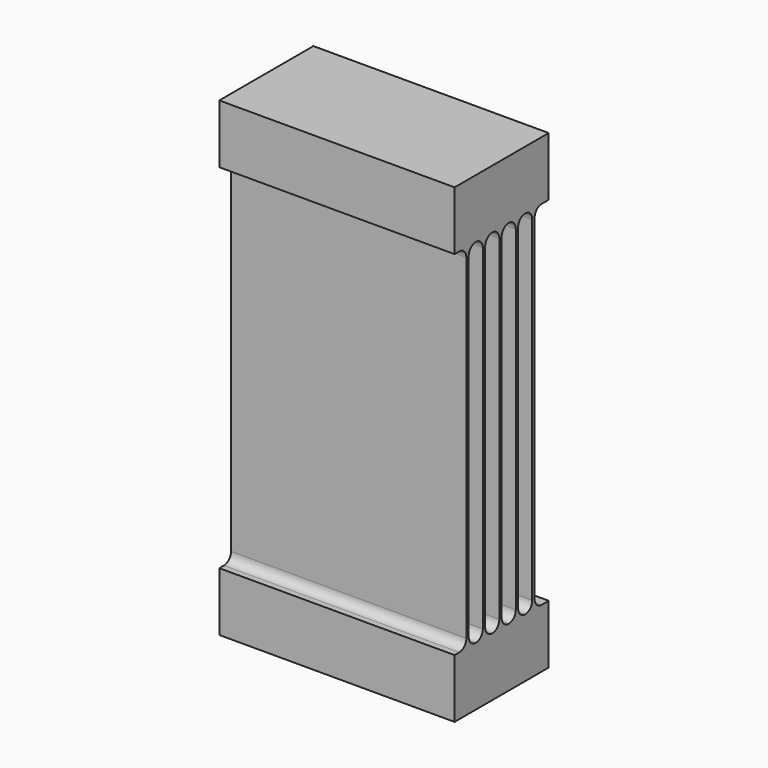
from build123d import *

# Parameters (mm, degrees)
F0_W     = 40
F0_H     = 20
F1_DEPTH = 10
F3_W     = 40
F3_H     = 0.5
F4_DEPTH = 30
F6_R     = 1.49999


# Not quite as in the source:
# - a fillet or chamfer is up to 0.001 mm smaller than in the source, because OpenCascade refuses the exact size


with BuildPart() as f1:
    # F0 (on Top) → F1 (new body)
    with BuildSketch(Plane.XY):
        with Locations((20, -10)):
            Rectangle(F0_W, F0_H)
    extrude(amount=F1_DEPTH)

    # F3 (on face) → F4 (join)
    with BuildSketch(Plane.XY.offset(10)):
        with Locations((20, -3.25)):
            Rectangle(F3_W, F3_H)
        with Locations((20, -6.75)):
            Rectangle(F3_W, F3_H)
        with Locations((20, -10.25)):
            Rectangle(F3_W, F3_H)
        with Locations((20, -13.75)):
            Rectangle(F3_W, F3_H)
        with Locations((20, -17.25)):
            Rectangle(F3_W, F3_H)
    extrude(amount=F4_DEPTH)

    # F5: F1 across face


with BuildPart() as f1_1:
    add(f1.part)
    add(f1.part.mirror(Plane(origin=(20, -17.25, 40), x_dir=(1, 0, 0), z_dir=(0, 0, 1))))

    # F6 (radius 1.5 in the source; OpenCascade refuses exactly that, so slightly less here)
    f6_edges = [f1_1.edges().sort_by_distance(p)[0] for p in [
        (20, -17, 70),
        (20, -13.5, 70),
        (20, -10, 70),
        (20, -6.5, 70),
        (20, -3, 70),
        (20, -3.5, 70),
        (20, -7, 70),
        (20, -10.5, 70),
        (20, -14, 70),
        (20, -17.5, 70),
        (20, -17.5, 10),
        (20, -14, 10),
        (20, -10.5, 10),
        (20, -7, 10),
        (20, -3.5, 10),
        (20, -17, 10),
        (20, -13.5, 10),
        (20, -10, 10),
        (20, -6.5, 10),
        (20, -3, 10),
    ]]
    fillet(f6_edges, radius=F6_R)


solid = f1_1.part
